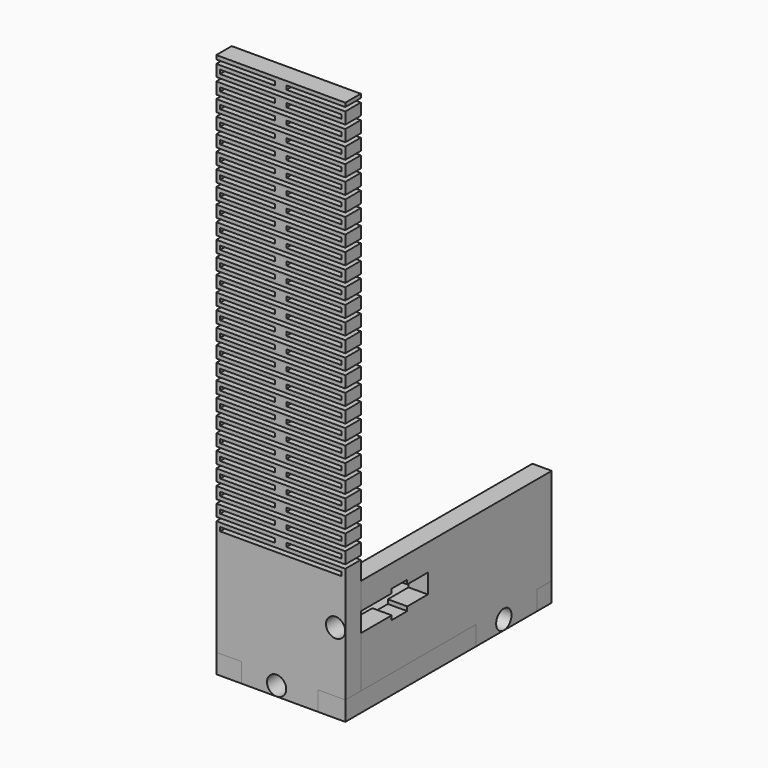
from build123d import *

# Parameters (mm, degrees)
F1_DEPTH = 3.81
F2_W     = 23.876
F2_H     = 0.762
F2_R     = 1.8923
F2_W_2   = 4.9914438277
F2_H_2   = 3.81
F3_DEPTH = 3.81
F4_D     = 3.7846
F5_R     = 1.8923
F6_DEPTH = 3.81


# Not quite as in the source:
# - a feature of the source that left no trace in its solid (it failed there, or was rolled back) is left out


with BuildPart() as f1:
    # F0 (on Top) → F1 (new body)
    with BuildSketch(Plane.XY):
        Polygon((-25.4, 0), (-25.4, -50.8), (-20.431529541, -50.8), (-20.431529541, -46.99), (-15.4400857132, -46.99), (-15.4400857132, -39.37), (-16.5662810173, -39.37), (-16.5662810173, -35.56), (-15.4400857132, -35.56), (-15.4400857132, -30.48), (-11.6300857132, -30.48), (-11.6300857132, -35.56), (-10.5038904092, -35.56), (-10.5038904092, -39.37), (-11.6300857132, -39.37), (-11.6300857132, -46.99), (-5.3635710352, -46.99), (-5.3635710352, -50.8), (0, -50.8), (0, -18.6903681606), (-3.81, -18.6903681606), (-3.81, -13.6989243329), (-11.43, -13.6989243329), (-11.43, -14.825119637), (-15.24, -14.825119637), (-15.24, -13.6989243329), (-20.32, -13.6989243329), (-20.32, -9.8889243329), (-15.24, -9.8889243329), (-15.24, -8.7627290288), (-11.43, -8.7627290288), (-11.43, -9.8889243329), (-3.81, -9.8889243329), (-3.81, -3.6224096548), (0, -3.6224096548), (0, 0), align=None)
    extrude(amount=F1_DEPTH)


with BuildPart() as f3:
    # F2 (on face) → F3 (new body)
    with BuildSketch(Plane.XZ.offset(46.99)):
        Polygon((-15.4400857132, 3.81), (-15.4400857132, 0), (-13.5194305331, 0), (-5.3635710352, 0), (-5.3635710352, 3.81), (0, 3.81), (0, 25.0114359447), (0, 26.5354359447), (-11.5787064001, 26.5354359447), (-11.5787064001, 27.2974359447), (0, 27.2974359447), (0, 28.0594359447), (0, 29.5834359447), (-11.5787064001, 29.5834359447), (-11.5787064001, 30.3454359447), (0, 30.3454359447), (0, 31.1074359447), (0, 32.6314359447), (-11.5787064001, 32.6314359447), (-11.5787064001, 33.3934359447), (0, 33.3934359447), (0, 34.1554359447), (0, 35.6794359447), (-11.5787064001, 35.6794359447), (-11.5787064001, 36.4414359447), (0, 36.4414359447), (0, 37.2034359447), (0, 38.7274359447), (-11.5787064001, 38.7274359447), (-11.5787064001, 39.4894359447), (0, 39.4894359447), (0, 40.2514359447), (0, 41.7754359447), (-11.5787064001, 41.7754359447), (-11.5787064001, 42.5374359447), (0, 42.5374359447), (0, 43.2994359447), (0, 44.8234359447), (-11.5787064001, 44.8234359447), (-11.5787064001, 45.5854359447), (0, 45.5854359447), (0, 46.3474359447), (0, 47.8714359447), (-11.5787064001, 47.8714359447), (-11.5787064001, 48.6334359447), (0, 48.6334359447), (0, 49.3954359447), (0, 50.9194359447), (-11.5787064001, 50.9194359447), (-11.5787064001, 51.6814359447), (0, 51.6814359447), (0, 52.4434359447), (0, 53.9674359447), (-11.5787064001, 53.9674359447), (-11.5787064001, 54.7294359447), (0, 54.7294359447), (0, 55.4914359447), (0, 57.0154359447), (-11.5787064001, 57.0154359447), (-11.5787064001, 57.7774359447), (0, 57.7774359447), (0, 58.5394359447), (0, 60.0634359447), (-11.5787064001, 60.0634359447), (-11.5787064001, 60.8254359447), (0, 60.8254359447), (0, 61.5874359447), (0, 63.1114359447), (-11.5787064001, 63.1114359447), (-11.5787064001, 63.8734359447), (0, 63.8734359447), (0, 64.6354359447), (0, 66.1594359447), (-11.5787064001, 66.1594359447), (-11.5787064001, 66.9214359447), (0, 66.9214359447), (0, 67.6834359447), (0, 69.2074359447), (-11.5787064001, 69.2074359447), (-11.5787064001, 69.9694359447), (0, 69.9694359447), (0, 70.7314359447), (0, 72.2554359447), (-11.5787064001, 72.2554359447), (-11.5787064001, 73.0174359447), (0, 73.0174359447), (0, 73.7794359447), (0, 75.3034359447), (-11.5787064001, 75.3034359447), (-11.5787064001, 76.0654359447), (0, 76.0654359447), (0, 76.8274359447), (0, 78.3514359447), (-11.5787064001, 78.3514359447), (-11.5787064001, 79.1134359447), (0, 79.1134359447), (0, 79.8754359447), (0, 81.3994359447), (-11.5787064001, 81.3994359447), (-11.5787064001, 82.1614359447), (0, 82.1614359447), (0, 82.9234359447), (0, 84.4474359447), (-11.5787064001, 84.4474359447), (-11.5787064001, 85.2094359447), (0, 85.2094359447), (0, 85.9714359447), (0, 87.4954359447), (-11.5787064001, 87.4954359447), (-11.5787064001, 88.2574359447), (0, 88.2574359447), (0, 89.0194359447), (0, 90.5434359447), (-11.5787064001, 90.5434359447), (-11.5787064001, 91.3054359447), (0, 91.3054359447), (0, 92.0674359447), (0, 93.5914359447), (-11.5787064001, 93.5914359447), (-11.5787064001, 94.3534359447), (0, 94.3534359447), (0, 95.1154359447), (0, 96.6394359447), (-11.5787064001, 96.6394359447), (-11.5787064001, 97.4014359447), (0, 97.4014359447), (0, 98.1634359447), (0, 99.6874359447), (-11.5787064001, 99.6874359447), (-11.5787064001, 100.4494359447), (0, 100.4494359447), (0, 101.2114359447), (0, 102.7354359447), (-11.5787064001, 102.7354359447), (-11.5787064001, 103.4974359447), (0, 103.4974359447), (0, 104.2594359447), (0, 105.7834359447), (-11.5787064001, 105.7834359447), (-11.5787064001, 106.5454359447), (0, 106.5454359447), (0, 107.3074359447), (-12.7, 107.3074359447), (-25.4, 107.3074359447), (-25.4, 106.5454359447), (-13.8212935999, 106.5454359447), (-13.8212935999, 105.7834359447), (-25.4, 105.7834359447), (-25.4, 104.2594359447), (-25.4, 103.4974359447), (-13.8212935999, 103.4974359447), (-13.8212935999, 102.7354359447), (-25.4, 102.7354359447), (-25.4, 101.2114359447), (-25.4, 100.4494359447), (-13.8212935999, 100.4494359447), (-13.8212935999, 99.6874359447), (-25.4, 99.6874359447), (-25.4, 98.1634359447), (-25.4, 97.4014359447), (-13.8212935999, 97.4014359447), (-13.8212935999, 96.6394359447), (-25.4, 96.6394359447), (-25.4, 95.1154359447), (-25.4, 94.3534359447), (-13.8212935999, 94.3534359447), (-13.8212935999, 93.5914359447), (-25.4, 93.5914359447), (-25.4, 92.0674359447), (-25.4, 91.3054359447), (-13.8212935999, 91.3054359447), (-13.8212935999, 90.5434359447), (-25.4, 90.5434359447), (-25.4, 89.0194359447), (-25.4, 88.2574359447), (-13.8212935999, 88.2574359447), (-13.8212935999, 87.4954359447), (-25.4, 87.4954359447), (-25.4, 85.9714359447), (-25.4, 85.2094359447), (-13.8212935999, 85.2094359447), (-13.8212935999, 84.4474359447), (-25.4, 84.4474359447), (-25.4, 82.9234359447), (-25.4, 82.1614359447), (-13.8212935999, 82.1614359447), (-13.8212935999, 81.3994359447), (-25.4, 81.3994359447), (-25.4, 79.8754359447), (-25.4, 79.1134359447), (-13.8212935999, 79.1134359447), (-13.8212935999, 78.3514359447), (-25.4, 78.3514359447), (-25.4, 76.8274359447), (-25.4, 76.0654359447), (-13.8212935999, 76.0654359447), (-13.8212935999, 75.3034359447), (-25.4, 75.3034359447), (-25.4, 73.7794359447), (-25.4, 73.0174359447), (-13.8212935999, 73.0174359447), (-13.8212935999, 72.2554359447), (-25.4, 72.2554359447), (-25.4, 70.7314359447), (-25.4, 69.9694359447), (-13.8212935999, 69.9694359447), (-13.8212935999, 69.2074359447), (-25.4, 69.2074359447), (-25.4, 67.6834359447), (-25.4, 66.9214359447), (-13.8212935999, 66.9214359447), (-13.8212935999, 66.1594359447), (-25.4, 66.1594359447), (-25.4, 64.6354359447), (-25.4, 63.8734359447), (-13.8212935999, 63.8734359447), (-13.8212935999, 63.1114359447), (-25.4, 63.1114359447), (-25.4, 61.5874359447), (-25.4, 60.8254359447), (-13.8212935999, 60.8254359447), (-13.8212935999, 60.0634359447), (-25.4, 60.0634359447), (-25.4, 58.5394359447), (-25.4, 57.7774359447), (-13.8212935999, 57.7774359447), (-13.8212935999, 57.0154359447), (-25.4, 57.0154359447), (-25.4, 55.4914359447), (-25.4, 54.7294359447), (-13.8212935999, 54.7294359447), (-13.8212935999, 53.9674359447), (-25.4, 53.9674359447), (-25.4, 52.4434359447), (-25.4, 51.6814359447), (-13.8212935999, 51.6814359447), (-13.8212935999, 50.9194359447), (-25.4, 50.9194359447), (-25.4, 49.3954359447), (-25.4, 48.6334359447), (-13.8212935999, 48.6334359447), (-13.8212935999, 47.8714359447), (-25.4, 47.8714359447), (-25.4, 46.3474359447), (-25.4, 45.5854359447), (-13.8212935999, 45.5854359447), (-13.8212935999, 44.8234359447), (-25.4, 44.8234359447), (-25.4, 43.2994359447), (-25.4, 42.5374359447), (-13.8212935999, 42.5374359447), (-13.8212935999, 41.7754359447), (-25.4, 41.7754359447), (-25.4, 40.2514359447), (-25.4, 39.4894359447), (-13.8212935999, 39.4894359447), (-13.8212935999, 38.7274359447), (-25.4, 38.7274359447), (-25.4, 37.2034359447), (-25.4, 36.4414359447), (-13.8212935999, 36.4414359447), (-13.8212935999, 35.6794359447), (-25.4, 35.6794359447), (-25.4, 34.1554359447), (-25.4, 33.3934359447), (-13.8212935999, 33.3934359447), (-13.8212935999, 32.6314359447), (-25.4, 32.6314359447), (-25.4, 31.1074359447), (-25.4, 30.3454359447), (-13.8212935999, 30.3454359447), (-13.8212935999, 29.5834359447), (-25.4, 29.5834359447), (-25.4, 28.0594359447), (-25.4, 27.2974359447), (-13.8212935999, 27.2974359447), (-13.8212935999, 26.5354359447), (-25.4, 26.5354359447), (-25.4, 25.0114359447), (-25.4, 3.81), (-20.431529541, 3.81), align=None)
        with BuildLine():
            ThreePointArc((-11.6144305331, 1.905), (-12.1723921149, 0.5579615818), (-13.5194305331, 0))
            ThreePointArc((-13.5194305331, 0), (-14.8664689512, 3.2520384182), (-11.6144305331, 1.905))
        make_face(mode=Mode.SUBTRACT)
        with Locations((-12.7, 25.3924359447)):
            Rectangle(F2_W, F2_H, mode=Mode.SUBTRACT)
        with Locations((-12.7, 28.4404359447)):
            Rectangle(F2_W, F2_H, mode=Mode.SUBTRACT)
        with Locations((-12.7, 31.4884359447)):
            Rectangle(F2_W, F2_H, mode=Mode.SUBTRACT)
        with Locations((-12.7, 34.5364359447)):
            Rectangle(F2_W, F2_H, mode=Mode.SUBTRACT)
        with Locations((-12.7, 37.5844359447)):
            Rectangle(F2_W, F2_H, mode=Mode.SUBTRACT)
        with Locations((-12.7, 40.6324359447)):
            Rectangle(F2_W, F2_H, mode=Mode.SUBTRACT)
        with Locations((-12.7, 43.6804359447)):
            Rectangle(F2_W, F2_H, mode=Mode.SUBTRACT)
        with Locations((-12.7, 46.7284359447)):
            Rectangle(F2_W, F2_H, mode=Mode.SUBTRACT)
        with Locations((-12.7, 49.7764359447)):
            Rectangle(F2_W, F2_H, mode=Mode.SUBTRACT)
        with Locations((-12.7, 52.8244359447)):
            Rectangle(F2_W, F2_H, mode=Mode.SUBTRACT)
        with Locations((-1.905, 15.7291591167)):
            Circle(F2_R, mode=Mode.SUBTRACT)
        with Locations((-12.7, 55.8724359447)):
            Rectangle(F2_W, F2_H, mode=Mode.SUBTRACT)
        with Locations((-12.7, 58.9204359447)):
            Rectangle(F2_W, F2_H, mode=Mode.SUBTRACT)
        with Locations((-12.7, 61.9684359447)):
            Rectangle(F2_W, F2_H, mode=Mode.SUBTRACT)
        with Locations((-12.7, 65.0164359447)):
            Rectangle(F2_W, F2_H, mode=Mode.SUBTRACT)
        with Locations((-12.7, 68.0644359447)):
            Rectangle(F2_W, F2_H, mode=Mode.SUBTRACT)
        with Locations((-12.7, 71.1124359447)):
            Rectangle(F2_W, F2_H, mode=Mode.SUBTRACT)
        with Locations((-12.7, 74.1604359447)):
            Rectangle(F2_W, F2_H, mode=Mode.SUBTRACT)
        with Locations((-12.7, 77.2084359447)):
            Rectangle(F2_W, F2_H, mode=Mode.SUBTRACT)
        with Locations((-12.7, 80.2564359447)):
            Rectangle(F2_W, F2_H, mode=Mode.SUBTRACT)
        with Locations((-12.7, 83.3044359447)):
            Rectangle(F2_W, F2_H, mode=Mode.SUBTRACT)
        with Locations((-12.7, 86.3524359447)):
            Rectangle(F2_W, F2_H, mode=Mode.SUBTRACT)
        with Locations((-12.7, 89.4004359447)):
            Rectangle(F2_W, F2_H, mode=Mode.SUBTRACT)
        with Locations((-12.7, 92.4484359447)):
            Rectangle(F2_W, F2_H, mode=Mode.SUBTRACT)
        with Locations((-12.7, 95.4964359447)):
            Rectangle(F2_W, F2_H, mode=Mode.SUBTRACT)
        with Locations((-12.7, 98.5444359447)):
            Rectangle(F2_W, F2_H, mode=Mode.SUBTRACT)
        with Locations((-12.7, 101.5924359447)):
            Rectangle(F2_W, F2_H, mode=Mode.SUBTRACT)
        with Locations((-12.7, 104.6404359447)):
            Rectangle(F2_W, F2_H, mode=Mode.SUBTRACT)
        with Locations((-17.9358076271, 1.905)):
            Rectangle(F2_W_2, F2_H_2)
        with BuildLine():
            ThreePointArc((-11.6144305331, 1.905), (-14.8664689512, 3.2520384182), (-13.5194305331, 0))
            ThreePointArc((-13.5194305331, 0), (-12.1723921149, 0.5579615818), (-11.6144305331, 1.905))
        make_face()
    extrude(amount=F3_DEPTH)

    # F4 (through all)
    with Locations(Plane(origin=(0, -46.99, 0), x_dir=(1, 0, 0), z_dir=(0, 1, 0))):
        with Locations((-13.5194305331, -1.905)):
            Hole(F4_D / 2)


with BuildPart() as f6:
    # F5 (on face) → F6 (new body)
    with BuildSketch(Plane.YZ):
        Polygon((-3.6224096548, 3.81), (0, 3.81), (0, 22.86), (-46.99, 22.86), (-46.99, 17.6341591167), (-39.37, 17.6341591167), (-39.37, 18.4547889886), (-35.56, 18.4547889886), (-35.56, 17.6341591167), (-30.48, 17.6341591167), (-30.48, 13.8241591167), (-35.56, 13.8241591167), (-35.56, 13.0035292449), (-39.37, 13.0035292449), (-39.37, 13.8241591167), (-46.99, 13.8241591167), (-46.99, 3.81), (-18.6903681606, 3.81), (-18.6903681606, 0), (-3.6224096548, 0), align=None)
        with Locations((-11.7939243329, 1.905)):
            Circle(F5_R, mode=Mode.SUBTRACT)
    extrude(amount=-F6_DEPTH)


solid = Compound([f1.part, f3.part, f6.part])
